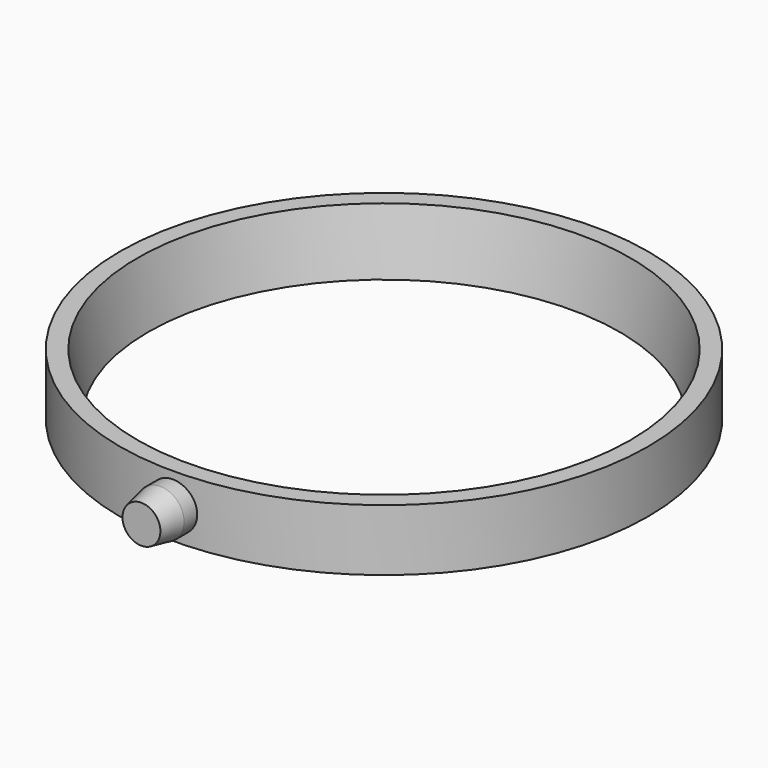
from build123d import *

# Parameters (mm, degrees)
F0_R     = 55.750000441
F0_R_2   = 49.75
F1_DEPTH = 13
F3_R     = 5
F4_DEPTH = 10
F5_SIZE2 = 2.292241
F5_SIZE  = 12.99999
F6_SIZE2 = 5
F6_SIZE  = 1


# Not quite as in the source:
# - a fillet or chamfer is up to 0.001 mm smaller than in the source, because OpenCascade refuses the exact size


with BuildPart() as f1:
    # F0 (on Top) → F1 (new body)
    with BuildSketch(Plane.XY):
        Circle(F0_R)
        Circle(F0_R_2, mode=Mode.SUBTRACT)
    extrude(amount=F1_DEPTH)

    # F3 (on offset) → F4 (join)
    with BuildSketch(Plane.XZ.offset(54)):
        with Locations((0, 6.4556576599)):
            Circle(F3_R)
    extrude(amount=F4_DEPTH)

    # F5 (size 13 and 2.2922507492 in the source; OpenCascade refuses exactly that, so slightly less here)
    f5_edges = [f1.edges().sort_by_distance(p)[0] for p in [
        (-49.75, 0, 13),
    ]]
    f5_side = f1.faces().sort_by_distance((-49.75, 0, 6.5))[0]
    chamfer(f5_edges, length=F5_SIZE, length2=F5_SIZE2, reference=f5_side)

    # F6
    f6_edges = [f1.edges().sort_by_distance(p)[0] for p in [
        (-5, -64, 6.455658),
    ]]
    f6_side = f1.faces().sort_by_distance((0, -64, 6.455658))[0]
    chamfer(f6_edges, length=F6_SIZE, length2=F6_SIZE2, reference=f6_side)


solid = f1.part
